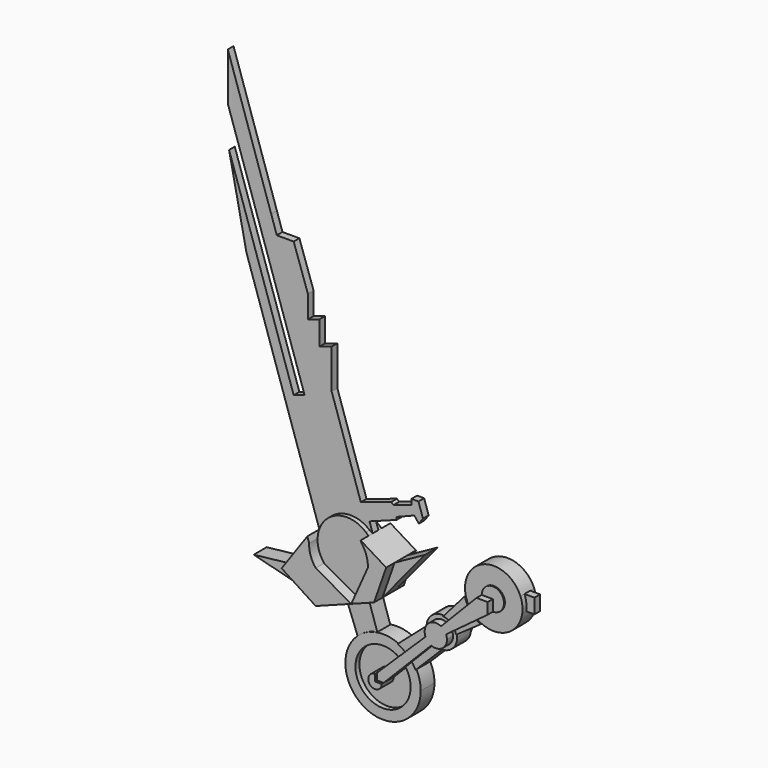
from build123d import *

# Parameters (mm, degrees)
F1_DEPTH = 1.27
F2_DEPTH = 1.3462
F3_DEPTH = 1.524
F4_DEPTH = 2.54
F5_DEPTH = 2.921
F6_DEPTH = 0.5588


with BuildPart() as f1:
    # F0 (on Front) → F1 (new body, symmetric)
    with BuildSketch(Plane.XZ):
        with BuildLine():
            ThreePointArc((-49.238688, 4.874512), (-49.008656, 3.22886), (-48.2102, 1.771618))
            Line((-48.2102, 1.771618), (-49.238688, 4.874512))
        make_face()
        with BuildLine():
            Line((-48.2102, 1.771618), (-42.631264, -1.356745))
            Line((-42.631264, -1.356745), (-40.025417, 4.484551))
            Line((-40.025417, 4.484551), (-41.053904, 7.587445))
            ThreePointArc((-41.053904, 7.587445), (-41.340663, 7.908443), (-41.656106, 8.2013))
            ThreePointArc((-41.656106, 8.2013), (-46.484528, 8.901787), (-49.238688, 4.874512))
            Line((-49.238688, 4.874512), (-48.2102, 1.771618))
        make_face()
        with BuildLine():
            Line((-41.053904, 7.587445), (-40.025417, 4.484551))
            ThreePointArc((-40.025417, 4.484551), (-40.255449, 6.130203), (-41.053904, 7.587445))
        make_face()
    extrude(amount=F1_DEPTH, both=True)


with BuildPart() as f1b:
    # F0 (on Front) → F1, piece 2 (new body, symmetric)
    with BuildSketch(Plane.XZ):
        Polygon((-37.1475, 5.438467), (-39.056565, 0), (-32.363176, 8.081837), align=None)
    extrude(amount=F1_DEPTH, both=True)


with BuildPart() as f1c:
    # F0 (on Front) → F1, piece 3 (new body, symmetric)
    with BuildSketch(Plane.XZ):
        Polygon((-59.259724, -0.638575), (-48.2102, -3.474181), (-53.555083, 0), align=None)
    extrude(amount=F1_DEPTH, both=True)


with BuildPart() as f1d:
    # F0 (on Front) → F1, piece 4 (new body, symmetric)
    with BuildSketch(Plane.XZ):
        with BuildLine():
            ThreePointArc((-42.958806, -6.564543), (-41.524521, -5.567995), (-39.861838, -5.033421))
            Line((-39.861838, -5.033421), (-41.240866, -0.829032))
            Line((-41.240866, -0.829032), (-42.631264, -1.356745))
            Line((-42.631264, -1.356745), (-44.645261, -2.12114))
            Line((-44.645261, -2.12114), (-42.958806, -6.564543))
        make_face()
    extrude(amount=F1_DEPTH, both=True)

    # F0 (on Front) → F2, piece 2 (join, symmetric)
    with BuildSketch(Plane.XZ):
        with BuildLine():
            ThreePointArc((-35.230178, -6.231052), (-35.833248, -5.812245), (-36.48353, -5.471326))
            ThreePointArc((-36.48353, -5.471326), (-38.140499, -5.004076), (-39.861838, -5.033421))
            ThreePointArc((-39.861838, -5.033421), (-41.524521, -5.567995), (-42.958806, -6.564543))
            ThreePointArc((-42.958806, -6.564543), (-41.24841, -16.307441), (-32.982495, -10.873825))
            ThreePointArc((-32.982495, -10.873825), (-33.152786, -9.464268), (-33.653859, -8.135819))
            ThreePointArc((-33.653859, -8.135819), (-33.930316, -7.66109), (-34.249598, -7.214038))
            Line((-34.249598, -7.214038), (-35.373487, -8.356668))
            ThreePointArc((-35.373487, -8.356668), (-34.773943, -9.552308), (-34.567542, -10.873825))
            ThreePointArc((-34.567542, -10.873825), (-42.75662, -12.853423), (-36.376024, -7.351805))
            Line((-36.376024, -7.351805), (-35.230178, -6.231052))
        make_face()
    extrude(amount=F2_DEPTH, both=True)


with BuildPart() as f2:
    # F0 (on Front) → F2 (new body, symmetric)
    with BuildSketch(Plane.XZ):
        with BuildLine():
            ThreePointArc((-17.008341, 5.604953), (-17.089608, 6.45769), (-17.330483, 7.279728))
            ThreePointArc((-17.330483, 7.279728), (-22.882389, 9.90992), (-25.916747, 4.568174))
            ThreePointArc((-25.916747, 4.568174), (-25.723954, 3.952091), (-25.445263, 3.369803))
            Line((-25.445263, 3.369803), (-23.273695, 5.604953))
            ThreePointArc((-23.273695, 5.604953), (-21.522875, 7.355772), (-19.772056, 5.604953))
            ThreePointArc((-19.772056, 5.604953), (-20.284859, 4.366936), (-21.522875, 3.854133))
            Line((-21.522875, 3.854133), (-24.131064, 1.920069))
            ThreePointArc((-24.131064, 1.920069), (-23.784129, 1.697556), (-23.418346, 1.507611))
            ThreePointArc((-23.418346, 1.507611), (-19.366394, 1.638769), (-17.053456, 4.968309))
            ThreePointArc((-17.053456, 4.968309), (-17.019634, 5.285832), (-17.008341, 5.604953))
        make_face()
    extrude(amount=F2_DEPTH, both=True)


with BuildPart() as f2b:
    # F0 (on Front) → F2, piece 3 (new body, symmetric)
    with BuildSketch(Plane.XZ):
        with BuildLine():
            ThreePointArc((-27.269002, -1.677323), (-27.279961, -1.448331), (-27.312738, -1.221432))
            ThreePointArc((-27.312738, -1.221432), (-27.397793, -0.902034), (-27.525962, -0.597367))
            Line((-27.525962, -0.597367), (-28.056798, -0.991001))
            ThreePointArc((-28.056798, -0.991001), (-27.952027, -1.327078), (-27.916625, -1.677323))
            ThreePointArc((-27.916625, -1.677323), (-28.712877, -3.144743), (-30.37716, -3.277028))
            Line((-30.37716, -3.277028), (-30.853346, -3.761155))
            ThreePointArc((-30.853346, -3.761155), (-30.242872, -4.005037), (-29.589109, -4.073972))
            ThreePointArc((-29.589109, -4.073972), (-27.944045, -3.345168), (-27.269002, -1.677323))
        make_face()
    extrude(amount=F2_DEPTH, both=True)


with BuildPart() as f2c:
    # F0 (on Front) → F2, piece 4 (new body, symmetric)
    with BuildSketch(Plane.XZ):
        with BuildLine():
            ThreePointArc((-28.381886, 0.347197), (-28.830562, 0.570007), (-29.315741, 0.694734))
            ThreePointArc((-29.315741, 0.694734), (-31.20602, 0.161461), (-32.063746, -1.605414))
            ThreePointArc((-32.063746, -1.605414), (-31.997092, -2.243225), (-31.763781, -2.840561))
            Line((-31.763781, -2.840561), (-31.27678, -2.364225))
            ThreePointArc((-31.27678, -2.364225), (-30.85119, -0.388528), (-28.846629, -0.131154))
            Line((-28.846629, -0.131154), (-28.381886, 0.347197))
        make_face()
    extrude(amount=F2_DEPTH, both=True)


with BuildPart() as f3:
    # F0 (on Front) → F3 (new body, symmetric)
    with BuildSketch(Plane.XZ):
        with BuildLine():
            ThreePointArc((-19.772056, 5.604953), (-21.522875, 7.355772), (-23.273695, 5.604953))
            Line((-23.273695, 5.604953), (-21.522875, 5.604953))
            Line((-21.522875, 5.604953), (-21.522875, 3.854133))
            ThreePointArc((-21.522875, 3.854133), (-20.284859, 4.366936), (-19.772056, 5.604953))
        make_face()
    extrude(amount=F3_DEPTH, both=True)


with BuildPart() as f3b:
    # F0 (on Front) → F3, piece 2 (new body, symmetric)
    with BuildSketch(Plane.XZ):
        with BuildLine():
            ThreePointArc((-25.445263, 3.369803), (-25.723954, 3.952091), (-25.916747, 4.568174))
            Line((-25.916747, 4.568174), (-29.315741, 0.694734))
            ThreePointArc((-29.315741, 0.694734), (-28.830562, 0.570007), (-28.381886, 0.347197))
            Line((-28.381886, 0.347197), (-25.445263, 3.369803))
        make_face()
    extrude(amount=F3_DEPTH, both=True)


with BuildPart() as f3c:
    # F0 (on Front) → F3, piece 3 (new body, symmetric)
    with BuildSketch(Plane.XZ):
        with BuildLine():
            Line((-27.312738, -1.221432), (-23.418346, 1.507611))
            ThreePointArc((-23.418346, 1.507611), (-23.784129, 1.697556), (-24.131064, 1.920069))
            Line((-24.131064, 1.920069), (-27.525962, -0.597367))
            ThreePointArc((-27.525962, -0.597367), (-27.397793, -0.902034), (-27.312738, -1.221432))
        make_face()
    extrude(amount=F3_DEPTH, both=True)


with BuildPart() as f3d:
    # F0 (on Front) → F3, piece 4 (new body, symmetric)
    with BuildSketch(Plane.XZ):
        with BuildLine():
            ThreePointArc((-31.763781, -2.840561), (-31.997092, -2.243225), (-32.063746, -1.605414))
            Line((-32.063746, -1.605414), (-36.48353, -5.471326))
            ThreePointArc((-36.48353, -5.471326), (-35.833248, -5.812245), (-35.230178, -6.231052))
            Line((-35.230178, -6.231052), (-31.763781, -2.840561))
        make_face()
    extrude(amount=F3_DEPTH, both=True)


with BuildPart() as f3e:
    # F0 (on Front) → F3, piece 5 (new body, symmetric)
    with BuildSketch(Plane.XZ):
        with BuildLine():
            Line((-33.653859, -8.135819), (-29.589109, -4.073972))
            ThreePointArc((-29.589109, -4.073972), (-30.242872, -4.005037), (-30.853346, -3.761155))
            Line((-30.853346, -3.761155), (-34.249598, -7.214038))
            ThreePointArc((-34.249598, -7.214038), (-33.930316, -7.66109), (-33.653859, -8.135819))
        make_face()
    extrude(amount=F3_DEPTH, both=True)


with BuildPart() as f4:
    # F0 (on Front) → F4 (new body, symmetric)
    with BuildSketch(Plane.XZ):
        with BuildLine():
            Line((-23.273695, 5.604953), (-25.445263, 3.369803))
            ThreePointArc((-25.445263, 3.369803), (-24.867653, 2.572878), (-24.131064, 1.920069))
            Line((-24.131064, 1.920069), (-21.522875, 3.854133))
            ThreePointArc((-21.522875, 3.854133), (-22.760892, 4.366936), (-23.273695, 5.604953))
        make_face()
        with BuildLine():
            Line((-21.522875, 5.604953), (-23.273695, 5.604953))
            ThreePointArc((-23.273695, 5.604953), (-22.760892, 4.366936), (-21.522875, 3.854133))
            Line((-21.522875, 3.854133), (-21.522875, 5.604953))
        make_face()
        with BuildLine():
            ThreePointArc((-24.131064, 1.920069), (-24.867653, 2.572878), (-25.445263, 3.369803))
            Line((-25.445263, 3.369803), (-28.381886, 0.347197))
            ThreePointArc((-28.381886, 0.347197), (-27.89001, -0.067169), (-27.525962, -0.597367))
            Line((-27.525962, -0.597367), (-24.131064, 1.920069))
        make_face()
        with BuildLine():
            ThreePointArc((-27.525962, -0.597367), (-27.89001, -0.067169), (-28.381886, 0.347197))
            Line((-28.381886, 0.347197), (-28.846629, -0.131154))
            ThreePointArc((-28.846629, -0.131154), (-28.377904, -0.493278), (-28.056798, -0.991001))
            Line((-28.056798, -0.991001), (-27.525962, -0.597367))
        make_face()
        with BuildLine():
            ThreePointArc((-28.056798, -0.991001), (-28.377904, -0.493278), (-28.846629, -0.131154))
            ThreePointArc((-28.846629, -0.131154), (-30.85119, -0.388528), (-31.27678, -2.364225))
            ThreePointArc((-31.27678, -2.364225), (-30.913522, -2.905929), (-30.37716, -3.277028))
            ThreePointArc((-30.37716, -3.277028), (-28.712877, -3.144743), (-27.916625, -1.677323))
            ThreePointArc((-27.916625, -1.677323), (-27.952027, -1.327078), (-28.056798, -0.991001))
        make_face()
        with BuildLine():
            ThreePointArc((-30.853346, -3.761155), (-31.371873, -3.363469), (-31.763781, -2.840561))
            Line((-31.763781, -2.840561), (-35.230178, -6.231052))
            ThreePointArc((-35.230178, -6.231052), (-34.710964, -6.693692), (-34.249598, -7.214038))
            Line((-34.249598, -7.214038), (-30.853346, -3.761155))
        make_face()
        with BuildLine():
            Line((-31.27678, -2.364225), (-31.763781, -2.840561))
            ThreePointArc((-31.763781, -2.840561), (-31.371873, -3.363469), (-30.853346, -3.761155))
            Line((-30.853346, -3.761155), (-30.37716, -3.277028))
            ThreePointArc((-30.37716, -3.277028), (-30.913522, -2.905929), (-31.27678, -2.364225))
        make_face()
        with BuildLine():
            ThreePointArc((-35.373487, -8.356668), (-35.833336, -7.812913), (-36.376024, -7.351805))
            Line((-36.376024, -7.351805), (-38.901351, -9.821833))
            ThreePointArc((-38.901351, -9.821833), (-38.157481, -10.129955), (-37.84936, -10.873825))
            Line((-37.84936, -10.873825), (-35.373487, -8.356668))
        make_face()
        with BuildLine():
            ThreePointArc((-34.249598, -7.214038), (-34.710964, -6.693692), (-35.230178, -6.231052))
            Line((-35.230178, -6.231052), (-36.376024, -7.351805))
            ThreePointArc((-36.376024, -7.351805), (-35.833336, -7.812913), (-35.373487, -8.356668))
            Line((-35.373487, -8.356668), (-34.249598, -7.214038))
        make_face()
        with BuildLine():
            ThreePointArc((-37.84936, -10.873825), (-38.157481, -10.129955), (-38.901351, -9.821833))
            Line((-38.901351, -9.821833), (-38.901351, -10.873825))
            Line((-38.901351, -10.873825), (-37.84936, -10.873825))
        make_face()
    extrude(amount=F4_DEPTH, both=True)


with BuildPart() as f5:
    # F0 (on Front) → F5 (new body, symmetric)
    with BuildSketch(Plane.XZ):
        with BuildLine():
            Line((-44.645261, -2.12114), (-42.631264, -1.356745))
            Line((-42.631264, -1.356745), (-48.2102, 1.771618))
            ThreePointArc((-48.2102, 1.771618), (-49.008656, 3.22886), (-49.238688, 4.874512))
            Line((-49.238688, 4.874512), (-49.524432, 5.736588))
            Line((-49.524432, 5.736588), (-53.555083, 0))
            Line((-53.555083, 0), (-48.2102, -3.474181))
            Line((-48.2102, -3.474181), (-44.645261, -2.12114))
        make_face()
    extrude(amount=F5_DEPTH, both=True)


with BuildPart() as f5b:
    # F0 (on Front) → F5, piece 2 (new body, symmetric)
    with BuildSketch(Plane.XZ):
        with BuildLine():
            Line((-42.631264, -1.356745), (-41.240866, -0.829032))
            Line((-41.240866, -0.829032), (-39.056565, 0))
            Line((-39.056565, 0), (-37.1475, 5.438467))
            Line((-37.1475, 5.438467), (-41.15574, 7.89468))
            Line((-41.15574, 7.89468), (-41.053904, 7.587445))
            ThreePointArc((-41.053904, 7.587445), (-40.255449, 6.130203), (-40.025417, 4.484551))
            Line((-40.025417, 4.484551), (-42.631264, -1.356745))
        make_face()
    extrude(amount=F5_DEPTH, both=True)


with BuildPart() as f5c:
    # F0 (on Front) → F5, piece 3 (new body, symmetric)
    with BuildSketch(Plane.XZ):
        with BuildLine():
            Line((-38.901351, -10.873825), (-38.901351, -9.821833))
            ThreePointArc((-38.901351, -9.821833), (-39.645222, -11.617696), (-37.84936, -10.873825))
            Line((-37.84936, -10.873825), (-38.901351, -10.873825))
        make_face()
    extrude(amount=F5_DEPTH, both=True)


with BuildPart() as f6:
    # F0 (on Front) → F6 (new body, symmetric)
    with BuildSketch(Plane.XZ):
        with BuildLine():
            Line((-38.901351, -9.821833), (-36.376024, -7.351805))
            ThreePointArc((-36.376024, -7.351805), (-42.75662, -12.853423), (-34.567542, -10.873825))
            ThreePointArc((-34.567542, -10.873825), (-34.773943, -9.552308), (-35.373487, -8.356668))
            Line((-35.373487, -8.356668), (-37.84936, -10.873825))
            ThreePointArc((-37.84936, -10.873825), (-39.645222, -11.617696), (-38.901351, -9.821833))
        make_face()
    extrude(amount=F6_DEPTH, both=True)


with BuildPart() as f6b:
    # F0 (on Front) → F6, piece 2 (new body, symmetric)
    with BuildSketch(Plane.XZ):
        with BuildLine():
            Line((-41.656106, 8.2013), (-41.15574, 7.89468))
            Line((-41.15574, 7.89468), (-41.656106, 9.40426))
            Line((-41.656106, 9.40426), (-37.395157, 10.978648))
            Line((-37.395157, 10.978648), (-37.395157, 11.40233))
            Line((-37.395157, 11.40233), (-34.625039, 12.494126))
            Line((-34.625039, 12.494126), (-33.908069, 11.597876))
            Line((-33.908069, 11.597876), (-33.26633, 12.512398))
            Line((-33.26633, 12.512398), (-33.973247, 14.645129))
            Line((-33.973247, 14.645129), (-35.075696, 14.645129))
            Line((-35.075696, 14.645129), (-35.075696, 13.826948))
            Line((-35.075696, 13.826948), (-37.868466, 12.901254))
            Line((-37.868466, 12.901254), (-38.254384, 13.181111))
            Line((-38.254384, 13.181111), (-43.014522, 11.603313))
            Line((-43.014522, 11.603313), (-47.597279, 25.429261))
            Line((-47.597279, 25.429261), (-47.597279, 31.616596))
            Line((-47.597279, 31.616596), (-49.531905, 30.975344))
            Line((-49.531905, 30.975344), (-49.531905, 34.750627))
            Line((-49.531905, 34.750627), (-51.329413, 34.154824))
            Line((-51.329413, 34.154824), (-51.329413, 37.700308))
            Line((-51.329413, 37.700308), (-53.555083, 44.192114))
            Line((-53.555083, 44.192114), (-56.205477, 44.192114))
            Line((-56.205477, 44.192114), (-57.086085, 46.848866))
            Line((-57.086085, 46.848866), (-63.891909, 67.381695))
            Line((-63.891909, 67.381695), (-63.891909, 59.880993))
            Line((-63.891909, 59.880993), (-51.843635, 23.531957))
            Line((-51.843635, 23.531957), (-53.555083, 22.964679))
            Line((-53.555083, 22.964679), (-63.694596, 53.555083))
            Line((-63.694596, 53.555083), (-60.969603, 40.266095))
            Line((-60.969603, 40.266095), (-49.524432, 5.736588))
            Line((-49.524432, 5.736588), (-49.238688, 4.874512))
            ThreePointArc((-49.238688, 4.874512), (-46.484528, 8.901787), (-41.656106, 8.2013))
        make_face()
    extrude(amount=F6_DEPTH, both=True)


with BuildPart() as f6c:
    # F0 (on Front) → F6, piece 3 (new body, symmetric)
    with BuildSketch(Plane.XZ):
        with BuildLine():
            Line((-15.762094, 4.968309), (-15.762094, 7.279728))
            Line((-15.762094, 7.279728), (-17.330483, 7.279728))
            ThreePointArc((-17.330483, 7.279728), (-17.089608, 6.45769), (-17.008341, 5.604953))
            ThreePointArc((-17.008341, 5.604953), (-17.019634, 5.285832), (-17.053456, 4.968309))
            Line((-17.053456, 4.968309), (-15.762094, 4.968309))
        make_face()
    extrude(amount=F6_DEPTH, both=True)


solid = Compound([f1.part, f1b.part, f1c.part, f1d.part, f2.part, f2b.part, f2c.part, f3.part, f3b.part, f3c.part, f3d.part, f3e.part, f4.part, f5.part, f5b.part, f5c.part, f6.part, f6b.part, f6c.part])
